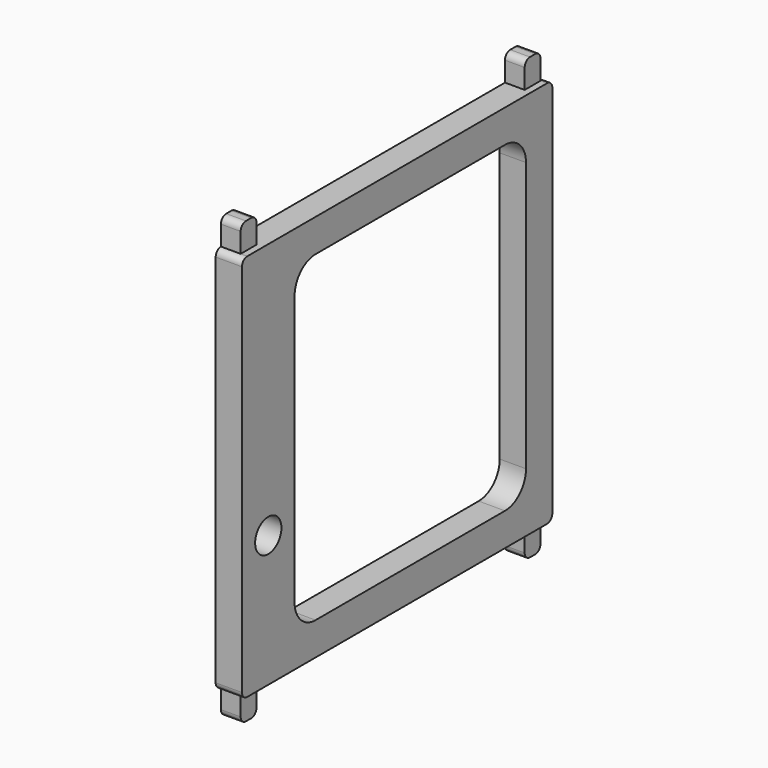
from build123d import *

# Parameters (mm, degrees)
F0_R     = 2.5
F0_W     = 3
F0_H     = 4
F1_DEPTH = 4
F2_W     = 3
F2_H     = 4
F3_DEPTH = 1
F4_R     = 4
F5_R     = 0.99999


# Not quite as in the source:
# - a fillet or chamfer is up to 0.001 mm smaller than in the source, because OpenCascade refuses the exact size


with BuildPart() as f1:
    # F0 (on Right) → F1 (new body)
    with BuildSketch(Plane.YZ):
        Polygon((-28.5, 29.5), (-29.5, 29.5), (-29.5, -29.5), (-28.5, -29.5), (-25.5, -29.5), (25.5, -29.5), (28.5, -29.5), (29.5, -29.5), (29.5, 29.5), (28.5, 29.5), (25.5, 29.5), (-25.5, 29.5), align=None)
        with Locations((-24.5, -9.5)):
            Circle(F0_R, mode=Mode.SUBTRACT)
        Polygon((19.5, -24.5), (-19.5, -24.5), (-19.5, 24.5), (19.5, 24.5), (24.5, 24.5), (24.5, -24.5), align=None, mode=Mode.SUBTRACT)
        with Locations((-27, 31.5)):
            Rectangle(F0_W, F0_H)
        with Locations((27, 31.5)):
            Rectangle(F0_W, F0_H)
        with Locations((-27, -31.5)):
            Rectangle(F0_W, F0_H)
        with Locations((27, -31.5)):
            Rectangle(F0_W, F0_H)
    extrude(amount=F1_DEPTH)

    # F2 (on face) → F3 (cut)
    with BuildSketch(Plane.YZ.offset(4)):
        with Locations((-27, 31.5)):
            Rectangle(F2_W, F2_H)
        with Locations((27, 31.5)):
            Rectangle(F2_W, F2_H)
        with Locations((-27, -31.5)):
            Rectangle(F2_W, F2_H)
        with Locations((27, -31.5)):
            Rectangle(F2_W, F2_H)
    extrude(amount=-F3_DEPTH, mode=Mode.SUBTRACT)

    # F4
    f4_edges = [f1.edges().sort_by_distance(p)[0] for p in [
        (2, -19.5, 24.5),
        (2, 24.5, 24.5),
        (2, 24.5, -24.5),
        (2, -19.5, -24.5),
    ]]
    fillet(f4_edges, radius=F4_R)

    # F5 (radius 1 in the source; OpenCascade refuses exactly that, so slightly less here)
    f5_edges = [f1.edges().sort_by_distance(p)[0] for p in [
        (1.5, -28.5, 33.5),
        (2, -29.5, 29.5),
        (1.5, -25.5, 33.5),
        (1.5, 25.5, 33.5),
        (1.5, 28.5, 33.5),
        (2, 29.5, 29.5),
        (1.5, -25.5, -33.5),
        (1.5, -28.5, -33.5),
        (2, -29.5, -29.5),
        (1.5, 25.5, -33.5),
        (1.5, 28.5, -33.5),
        (2, 29.5, -29.5),
    ]]
    fillet(f5_edges, radius=F5_R)


solid = f1.part
